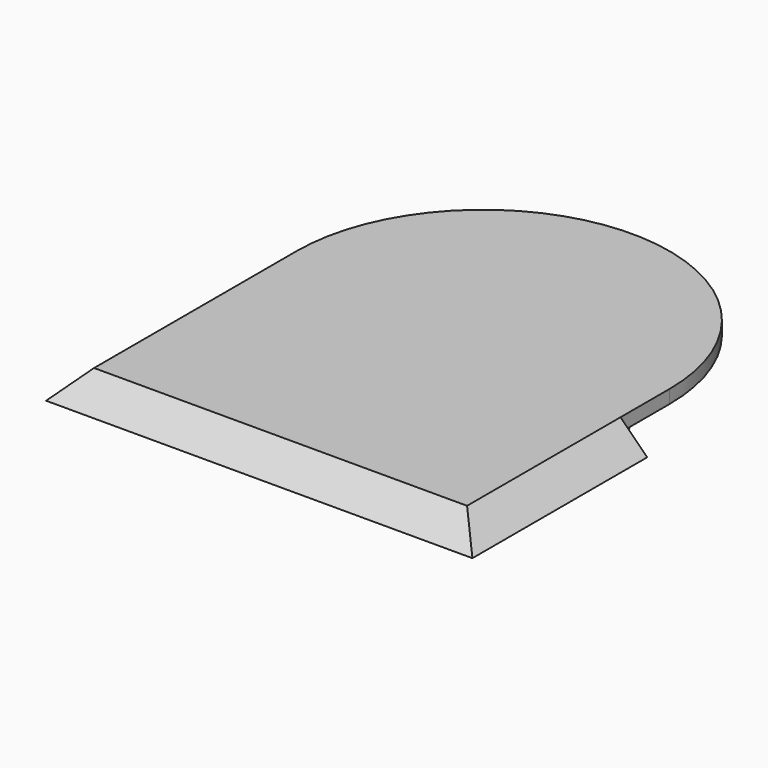
from build123d import *

# Parameters (mm, degrees)
F1_DEPTH = 5
F2_SIZE  = 4.99999
F4_DEPTH = 2.5


# Not quite as in the source:
# - a fillet or chamfer is up to 0.001 mm smaller than in the source, because OpenCascade refuses the exact size


with BuildPart() as f1:
    # F0 (on Top) → F1 (new body)
    with BuildSketch(Plane.XY):
        Polygon((-35, -47.5), (35, -47.5), (35, -11.5), (24.9973740429, 8.3822524399), (14.7012080997, -26.056649141), (0, 0), (-10.1516069844, -11.1895399168), (-20.0927332044, 15.4384765774), (-35, -14.7399436682), align=None)
        Polygon((35, -11.5), (35, -47.5), (-35, -47.5), (-35, -14.7399436682), (-40, -14.7399436682), (-40, -52.5), (40, -52.5), (40, -11.5), align=None)
    extrude(amount=F1_DEPTH)

    # F2 (size 5 in the source; OpenCascade refuses exactly that, so slightly less here)
    f2_edges = [f1.edges().sort_by_distance(p)[0] for p in [
        (-40, -33.619972, 5),
        (0, -52.5, 5),
        (40, -32, 5),
    ]]
    chamfer(f2_edges, length=F2_SIZE)

    # F3 (on face) → F4 (join)
    with BuildSketch(Plane.XY.offset(5)):
        Polygon((14.7012080997, -26.056649141), (18.0845528677, -14.7399436682), (8.3163026095, -14.7399436682), align=None)
        with BuildLine():
            ThreePointArc((33.7950026252, -9.1048227638), (34.6974429309, -4.5921078013), (35, 0))
            ThreePointArc((35, 0), (0, 35), (-35, 0))
            ThreePointArc((-35, 0), (-34.5462471197, -5.6175448326), (-33.1967537173, -11.0894338283))
            Line((-33.1967537173, -11.0894338283), (-20.0927332044, 15.4384765774))
            Line((-20.0927332044, 15.4384765774), (-10.1516069844, -11.1895399168))
            Line((-10.1516069844, -11.1895399168), (0, 0))
            Line((0, 0), (8.3163026095, -14.7399436682))
            Line((8.3163026095, -14.7399436682), (18.0845528677, -14.7399436682))
            Line((18.0845528677, -14.7399436682), (24.9973740429, 8.3822524399))
            Line((24.9973740429, 8.3822524399), (33.7950026252, -9.1048227638))
        make_face()
        with BuildLine():
            Line((35, -11.5), (35, 0))
            ThreePointArc((35, 0), (34.6974429309, -4.5921078013), (33.7950026252, -9.1048227638))
            Line((33.7950026252, -9.1048227638), (35, -11.5))
        make_face()
        with BuildLine():
            ThreePointArc((-33.1967537173, -11.0894338283), (-34.5462471197, -5.6175448326), (-35, 0))
            Line((-35, 0), (-35, -14.7399436682))
            Line((-35, -14.7399436682), (-33.1967537173, -11.0894338283))
        make_face()
    extrude(amount=-F4_DEPTH)


solid = f1.part
